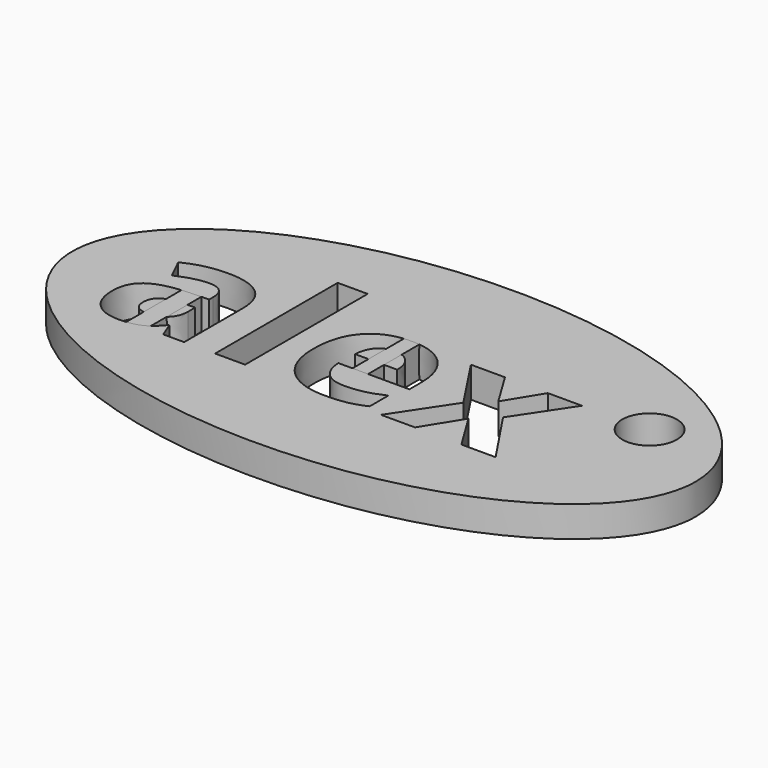
from build123d import *

# Parameters (mm, degrees)
F1_DEPTH     = 8
F2_R         = 7.0938880629
F2_TEXT_SIZE = 52.3472101324
F3_DEPTH     = 25
F5_DEPTH     = 8


# Not quite as in the source:
# - Text() gives the source's letters only with a copy of the font that has no kerning and outlines rounded to 1/6400 em; it was checked with that copy


with BuildPart() as f1:
    # F0 (on Top) → F1 (new body)
    with BuildSketch(Plane.XY):
        with BuildLine():
            add(Edge.make_bspline(
                [(51.104025382, 0), (51.104025382, 73.4083834691), (-70.2913317026, 36.7041917346), (-191.6866887871, 0), (-70.2913317026, -36.7041917346), (51.104025382, -73.4083834691), (51.104025382, 0)],
                knots=[0, 0, 0, 2.0943951024, 2.0943951024, 4.1887902048, 4.1887902048, 6.2831853072, 6.2831853072, 6.2831853072], degree=2, weights=[1, 0.5, 1, 0.5, 1, 0.5, 1]))
        make_face()
    extrude(amount=F1_DEPTH)

    # F2 (on face) → F3 (cut)
    with BuildSketch(Plane.XY.offset(8)):
        with Locations((29.4890962541, 12.0251402259)):
            Circle(F2_R)
        with Locations((-95.8300400525, -16.9652346522)):
            Text('alex', F2_TEXT_SIZE, font='Open Sans', font_style=FontStyle.BOLD, text_align=(TextAlign.LEFT, TextAlign.BOTTOM))
    extrude(amount=-F3_DEPTH, mode=Mode.SUBTRACT)


with BuildPart() as f5:
    # F4 (on face) → F5 (new body, through all)
    with BuildSketch(Plane.XY.offset(8)):
        with BuildLine():
            add(Edge.make_bspline(
                [(-30.2869342268, 12.0352423382), (-31.2804589665, 12.1447217324), (-33.3777527381, 12.1447217324), (-34.3254804611, 12.0434312847)],
                knots=[1.8217988017, 1.8217988017, 1.8217988017, 2, 2.168307372, 2.168307372, 2.168307372], degree=2))
            Line((-34.3254804611, 12.0434312847), (-34.3254804611, -4.6227440131))
            Line((-34.3254804611, -4.6227440131), (-30.2869342268, -4.6227440131))
            Line((-30.2869342268, -4.6227440131), (-30.2869342268, 12.0352423382))
        make_face()
    extrude(amount=-F5_DEPTH)


with BuildPart() as f5b:
    # F4 (on face) → F5, piece 2 (new body, through all)
    with BuildSketch(Plane.XY.offset(8)):
        with BuildLine():
            add(Edge.make_bspline(
                [(-80.8538304037, 0.6692317612), (-81.890814851, 0.6321966024), (-82.843311131, 0.5446824373)],
                knots=[0, 0, 0, 0.1617121359, 0.1617121359, 0.1617121359], degree=2))
            Line((-82.843311131, 0.5446824373), (-82.843311131, -17.3890048963))
            add(Edge.make_bspline(
                [(-82.843311131, -17.3890048963), (-80.799097715, -17.1839488379), (-78.5990510807, -16.1702018594), (-77.8572782874, -15.6205551182)],
                knots=[4.149714267, 4.149714267, 4.149714267, 4.6866320065, 4.968844946, 4.968844946, 4.968844946], degree=2))
            Line((-77.8572782874, -15.6205551182), (-77.8572782874, 0.7630282854))
            Line((-77.8572782874, 0.7630282854), (-80.8538304037, 0.6692317612))
        make_face()
    extrude(amount=-F5_DEPTH)


solid = Compound([f1.part, f5.part, f5b.part])
